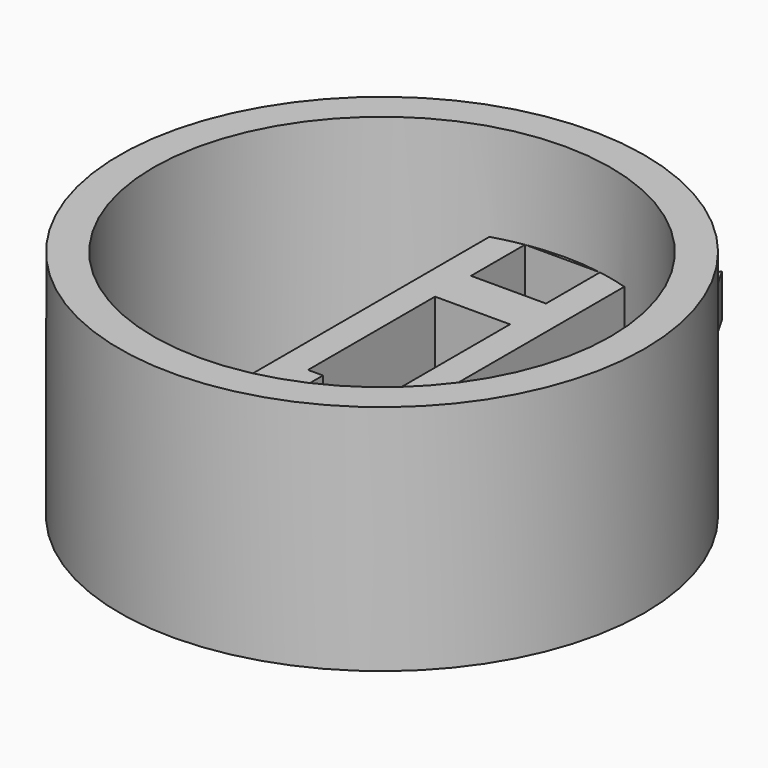
from build123d import *

# Parameters (mm, degrees)
F0_R     = 35
F0_W     = 2
F0_H     = 3
F1_DEPTH = 18
F2_R     = 35
F2_R_2   = 30.5
F3_DEPTH = 31
F5_DEPTH = 5.7


with BuildPart() as f1:
    # F0 (on Top) → F1 (new body)
    with BuildSketch(Plane.XY):
        Circle(F0_R)
        with BuildLine():
            ThreePointArc((-5, 30.0873727667), (0, 30.5), (5, 30.0873727667))
            Line((5, 30.0873727667), (9, 30.0873727667))
            Line((9, 30.0873727667), (9, 29.1418942418))
            ThreePointArc((9, 29.1418942418), (24.5433290325, 18.1073189622), (30.5, 0))
            ThreePointArc((30.5, 0), (24.5433290325, -18.1073189622), (9, -29.1418942418))
            ThreePointArc((9, -29.1418942418), (7.0159448694, -29.6820908561), (5, -30.0873727667))
            ThreePointArc((5, -30.0873727667), (0, -30.5), (-5, -30.0873727667))
            Line((-5, -30.0873727667), (-9, -30.0876272333))
            Line((-9, -30.0876272333), (-9, -29.1418942418))
            ThreePointArc((-9, -29.1418942418), (-30.5, 0), (-9, 29.1418942418))
            Line((-9, 29.1418942418), (-9, 30.0873727667))
            Line((-9, 30.0873727667), (-5, 30.0873727667))
        make_face(mode=Mode.SUBTRACT)
        with BuildLine():
            Line((-5, 30.0873727667), (5, 30.0873727667))
            ThreePointArc((5, 30.0873727667), (0, 30.5), (-5, 30.0873727667))
        make_face()
        with BuildLine():
            Line((9, 30.0873727667), (5, 30.0873727667))
            ThreePointArc((5, 30.0873727667), (7.0159448694, 29.6820908561), (9, 29.1418942418))
            Line((9, 29.1418942418), (9, 30.0873727667))
        make_face()
        with BuildLine():
            ThreePointArc((9, 29.1418942418), (7.0159448694, 29.6820908561), (5, 30.0873727667))
            Line((5, 30.0873727667), (5, 21.0873727667))
            Line((5, 21.0873727667), (5, 15.0873727667))
            Line((5, 15.0873727667), (5, -6.0873727667))
            Line((5, -6.0873727667), (5, -9.0873727667))
            Line((5, -9.0873727667), (5, -14.0873727667))
            Line((5, -14.0873727667), (5, -30.0873727667))
            ThreePointArc((5, -30.0873727667), (7.0159448694, -29.6820908561), (9, -29.1418942418))
            Line((9, -29.1418942418), (9, 29.1418942418))
        make_face()
        with BuildLine():
            Line((-5, 21.0873727667), (-5, 30.0873727667))
            ThreePointArc((-5, 30.0873727667), (-7.0159448694, 29.6820908561), (-9, 29.1418942418))
            Line((-9, 29.1418942418), (-9, -29.1418942418))
            ThreePointArc((-9, -29.1418942418), (-7.0159448694, -29.6820908561), (-5, -30.0873727667))
            Line((-5, -30.0873727667), (-5, -14.0873727667))
            Line((-5, -14.0873727667), (-5, -9.0873727667))
            Line((-5, -9.0873727667), (-5, -6.0873727667))
            Line((-5, -6.0873727667), (-5, 15.0873727667))
            Line((-5, 15.0873727667), (-5, 21.0873727667))
        make_face()
        with BuildLine():
            ThreePointArc((-9, 29.1418942418), (-7.0159448694, 29.6820908561), (-5, 30.0873727667))
            Line((-5, 30.0873727667), (-9, 30.0873727667))
            Line((-9, 30.0873727667), (-9, 29.1418942418))
        make_face()
        Polygon((5, 15.0873727667), (5, 21.0873727667), (0, 21.0873727667), (-5, 21.0873727667), (-5, 15.0873727667), (0, 15.0873727667), align=None)
        with BuildLine():
            ThreePointArc((-5, -30.0873727667), (-7.0159448694, -29.6820908561), (-9, -29.1418942418))
            Line((-9, -29.1418942418), (-9, -30.0876272333))
            Line((-9, -30.0876272333), (-5, -30.0873727667))
        make_face()
        with BuildLine():
            ThreePointArc((-5, -30.0873727667), (0, -30.5), (5, -30.0873727667))
            Line((5, -30.0873727667), (-5, -30.0873727667))
        make_face()
        with Locations((4, -7.5873727667)):
            Rectangle(F0_W, F0_H)
        with Locations((-4, -7.5873727667)):
            Rectangle(F0_W, F0_H)
        Polygon((0, -14.0873727667), (5, -14.0873727667), (5, -9.0873727667), (3, -9.0873727667), (0, -9.0873727667), (-3, -9.0873727667), (-5, -9.0873727667), (-5, -14.0873727667), align=None)
    extrude(amount=F1_DEPTH)

    # F2 (on Top) → F3 (join)
    with BuildSketch(Plane.XY):
        Circle(F2_R)
        Circle(F2_R_2, mode=Mode.SUBTRACT)
    extrude(amount=F3_DEPTH)

    # F4 (on Top) → F5 (join)
    with BuildSketch(Plane.XY):
        with BuildLine():
            ThreePointArc((-14.2633631023, 31.9617970867), (0, 35), (14.2633631023, 31.9617970867))
            Line((14.2633631023, 31.9617970867), (0, 56.6666666667))
            Line((0, 56.6666666667), (-14.2633631023, 31.9617970867))
        make_face()
    extrude(amount=F5_DEPTH)


solid = f1.part
